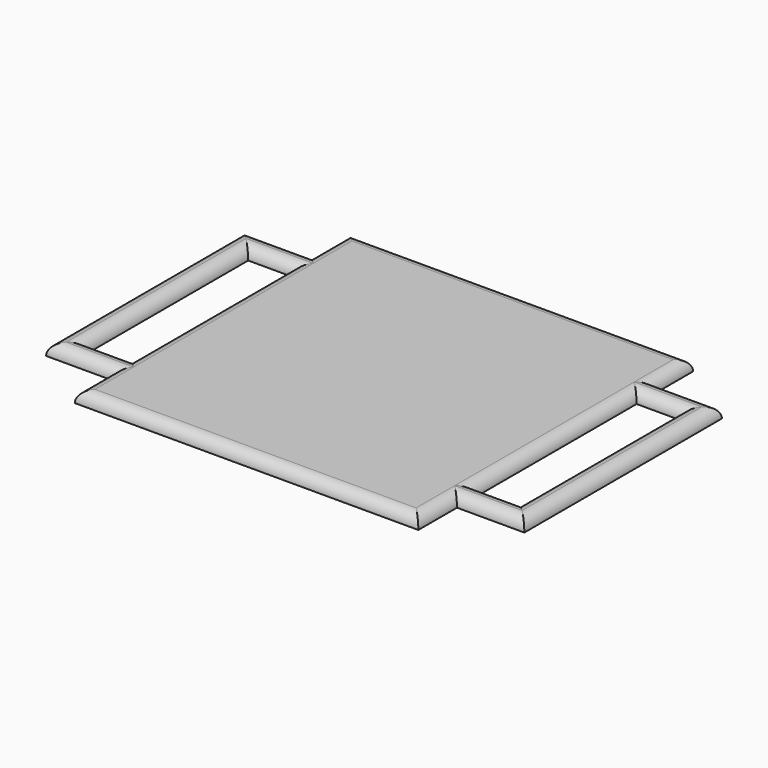
from build123d import *

# Parameters (mm, degrees)
F2_DEPTH = 5
F3_R     = 4.99999


# Not quite as in the source:
# - a fillet or chamfer is up to 0.001 mm smaller than in the source, because OpenCascade refuses the exact size


with BuildPart() as f2:
    # F1 (on Top) → F2 (new body)
    with BuildSketch(Plane.XY):
        Polygon((-76.5, -76.5), (76.5, -76.5), (76.5, -55), (76.5, -45), (76.5, 45), (76.5, 55), (76.5, 76.5), (-76.5, 76.5), (-76.5, 55), (-76.5, 45), (-76.5, -45), (-76.5, -55), align=None)
        Polygon((76.5, -45), (76.5, -55), (106.5, -55), (106.5, 55), (76.5, 55), (76.5, 45), (96.5, 45), (96.5, -45), align=None)
        Polygon((-106.5, -55), (-76.5, -55), (-76.5, -45), (-96.5, -45), (-96.5, 45), (-76.5, 45), (-76.5, 55), (-106.5, 55), align=None)
    extrude(amount=F2_DEPTH)

    # F3 (radius 5 in the source; OpenCascade refuses exactly that, so slightly less here)
    f3_edges = [f2.edges().sort_by_distance(p)[0] for p in [
        (0, -76.5, 5),
        (76.5, -65.75, 5),
        (91.5, -55, 5),
        (106.5, 0, 5),
        (91.5, 55, 5),
        (76.5, 65.75, 5),
        (0, 76.5, 5),
        (-76.5, 65.75, 5),
        (-91.5, 55, 5),
        (-106.5, 0, 5),
        (-91.5, -55, 5),
        (-76.5, -65.75, 5),
        (-76.5, 0, 5),
        (-86.5, -45, 5),
        (-96.5, 0, 5),
        (-86.5, 45, 5),
        (76.5, 0, 5),
        (86.5, 45, 5),
        (96.5, 0, 5),
        (86.5, -45, 5),
    ]]
    fillet(f3_edges, radius=F3_R)


solid = f2.part
